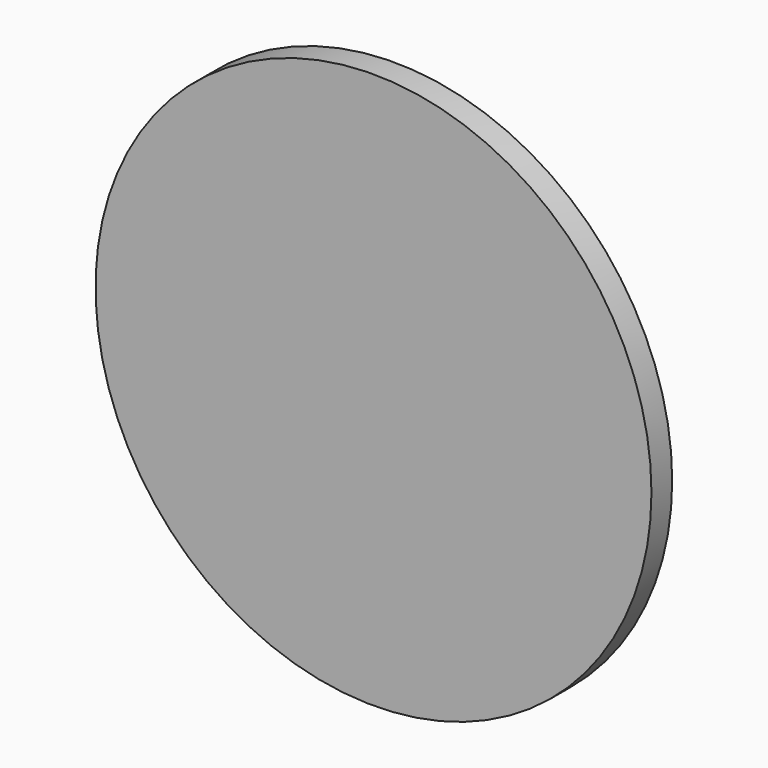
from build123d import *

# Parameters (mm, degrees)
F0_R     = 53.6264206078
F1_DEPTH = 2.5


# Not quite as in the source:
# - a feature of the source that left no trace in its solid (it failed there, or was rolled back) is left out


with BuildPart() as f1:
    # F0 (on Front) → F1 (new body, symmetric)
    with BuildSketch(Plane.XZ):
        with Locations((2.8825884219, 0)):
            Circle(F0_R)
    extrude(amount=F1_DEPTH, both=True)


solid = f1.part
